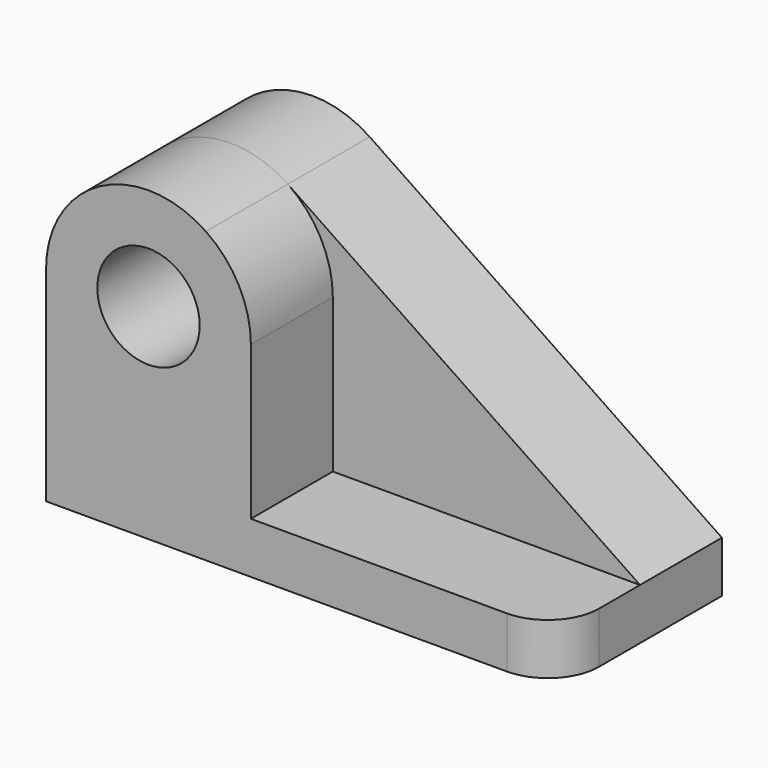
from build123d import *

# Parameters (mm, degrees)
F0_R     = 12.7
F1_DEPTH = 25.4
F2_R     = 12.7
F3_DEPTH = 25.4
F4_R     = 12.7


# Not quite as in the source:
# - ends of sketch curves that miss each other by under 0.0002 mm in the source are joined


with BuildPart() as f1:
    # F0 (on Front) → F1 (new body)
    with BuildSketch(Plane.XZ):
        with BuildLine():
            Line((44.2728957302, 3.7863082206), (-43.0928697159, 62.9011237785))
            ThreePointArc((-43.0928697159, 62.9011237785), (-69.2256049206, 64.3050592902), (-82.7271042698, 41.8863082206))
            ThreePointArc((-82.7271042698, 41.8863082206), (-82.7271113952, 41.8753238207), (-82.7271137703, 41.8643394188))
            Line((-82.7271137703, 41.8643394188), (-82.7271042698, -8.9136917794))
            Line((-82.7271042698, -8.9136917794), (44.2728957302, -8.9136917794))
            Line((44.2728957302, -8.9136917794), (44.2728957302, 3.7863082206))
        make_face()
        with Locations((-57.3271137703, 41.8643394188)):
            Circle(F0_R, mode=Mode.SUBTRACT)
    extrude(amount=F1_DEPTH)

    # F2 (on face) → F3 (join)
    with BuildSketch(Plane.XZ.offset(25.4)):
        with BuildLine():
            Line((-31.9271232709, 3.7863082206), (-31.9271232709, 41.8643394188))
            ThreePointArc((-31.9271232709, 41.8643394188), (-34.8915499721, 53.7725296435), (-43.0928750401, 62.90111591))
            ThreePointArc((-43.0928750401, 62.90111591), (-69.2256004701, 64.3050508965), (-82.7270947692, 41.8863082124))
            ThreePointArc((-82.7270947692, 41.8863082124), (-82.7271018946, 41.8753238166), (-82.7271042698, 41.8643394188))
            Line((-82.7271042698, 41.8643394188), (-82.7271042698, 3.7863082206))
            Line((-82.7271042698, 3.7863082206), (-82.7271042698, -8.9136917794))
            Line((-82.7271042698, -8.9136917794), (44.2728957302, -8.9136917794))
            Line((44.2728957302, -8.9136917794), (44.2728957302, 3.7863082206))
            Line((44.2728957302, 3.7863082206), (-31.9271232709, 3.7863082206))
        make_face()
        with Locations((-57.3271137703, 41.8643394188)):
            Circle(F2_R, mode=Mode.SUBTRACT)
    extrude(amount=F3_DEPTH)

    # F4
    f4_edges = [f1.edges().sort_by_distance(p)[0] for p in [
        (44.272896, -50.8, -2.563692),
    ]]
    fillet(f4_edges, radius=F4_R)


solid = f1.part
